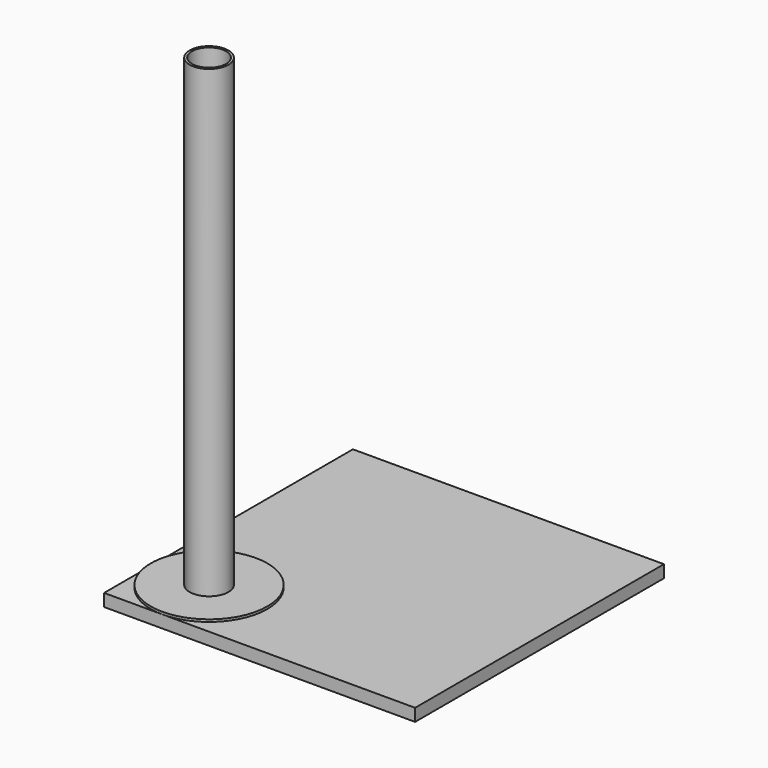
from build123d import *

# Parameters (mm, degrees)
F0_R     = 25
F1_DEPTH = 600
F2_T     = -3
F3_R     = 75
F4_DEPTH = 3
F5_W     = 400
F5_H     = 400
F6_DEPTH = 16


# Not quite as in the source:
# - a feature names something its author has since deleted; it is built from what else it names


with BuildPart() as f1:
    # F0 (on Top) → F1 (new body)
    with BuildSketch(Plane.XY):
        Circle(F0_R)
    extrude(amount=F1_DEPTH)

    # F2
    f2_openings = [f1.faces().sort_by_distance(p)[0] for p in [
        (0, 0, 600),
        (0, 0, 0),
    ]]
    offset(amount=F2_T, openings=f2_openings)

    # F3 (on Top) → F4 (join)
    with BuildSketch(Plane.XY):
        Circle(F3_R)
    extrude(amount=F4_DEPTH)

    # F5 (on Top) → F6 (join)
    with BuildSketch(Plane.XY):
        with Locations((125, 125)):
            Rectangle(F5_W, F5_H)
    extrude(amount=-F6_DEPTH)


solid = f1.part
